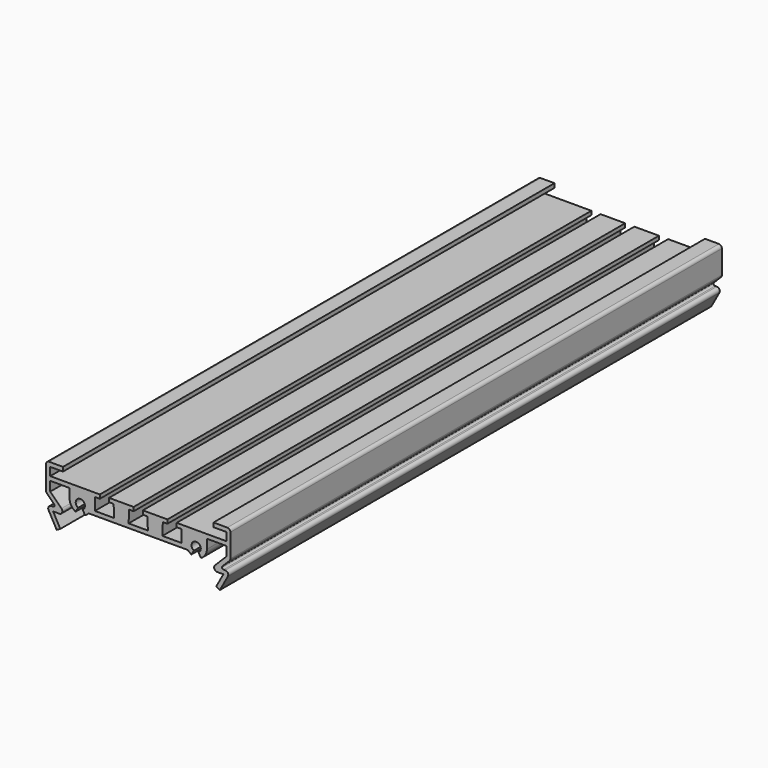
from build123d import *

# Parameters (mm, degrees)
F1_DEPTH = 200


# Not quite as in the source:
# - ends of sketch curves that miss each other by under 0.0002 mm in the source are joined


with BuildPart() as f1:
    # F0 (on Front) → F1 (new body)
    with BuildSketch(Plane.XZ):
        with BuildLine():
            Line((-18.103784, -0.791851), (-17.32476, -2.14116))
            ThreePointArc((-17.32476, -2.14116), (-16.7014064944, -1.7527534112), (-16.1728328101, -1.2428131594))
            Line((-16.1728328101, -1.2428131594), (16.172833, -1.242813))
            ThreePointArc((16.172833, -1.242813), (16.7014064944, -1.7527534112), (17.3247602013, -2.1411595856))
            Line((17.3247602013, -2.1411595856), (18.103784, -0.791851))
            ThreePointArc((18.103784, -0.791851), (18.853784, 2.007187), (19.6037840458, -0.7918510793))
            Line((19.6037840458, -0.7918510793), (20.382808, -2.14116))
            ThreePointArc((20.382808, -2.14116), (21.820396824, -0.8500174455), (22.353784, 1.007187))
            Line((22.353784, 1.007187), (22.353784, 4.007187))
            Line((22.353784, 4.007187), (28.65, 4.007187))
            Line((28.65, 4.007187), (28.65, 0.916375))
            Line((28.65, 0.916375), (24.995488, -2.738136))
            ThreePointArc((24.995488, -2.738136), (24.7787154675, -3.8279264324), (25.702595, -4.445243))
            Line((25.702595, -4.445243), (27.714112, -4.445243))
            Line((27.714112, -4.445243), (25.365346, -8.705386))
            Line((25.365346, -8.705386), (26.54757, -9.357187))
            Line((26.54757, -9.357187), (29.182471, -4.578059))
            ThreePointArc((29.182471, -4.578059), (29.1678006221, -3.5867237514), (28.30675, -3.095243))
            Line((28.30675, -3.095243), (27.754677, -3.095243))
            ThreePointArc((27.754677, -3.095243), (27.292737369, -2.7865850428), (27.4011231094, -2.2416901094))
            Line((27.4011231094, -2.2416901094), (29.707107, 0.064294))
            ThreePointArc((29.707107, 0.064294), (29.9238795325, 0.3887175676), (30, 0.771401))
            Line((30, 0.771401), (30, 8.357187))
            ThreePointArc((30, 8.357187), (29.7071067812, 9.0642937812), (29, 9.357187))
            Line((29, 9.357187), (24.5, 9.357187))
            Line((24.5, 9.357187), (24.5, 8.007187))
            Line((24.5, 8.007187), (28.65, 8.007187))
            Line((28.65, 8.007187), (28.65, 5.357187))
            Line((28.65, 5.357187), (12.5, 5.357187))
            Line((12.5, 5.357187), (12.5, 4.107187))
            Line((12.5, 4.107187), (14, 4.107187))
            Line((14, 4.107187), (14.125, 0.107187))
            Line((14.125, 0.107187), (7.875, 0.107187))
            Line((7.875, 0.107187), (8, 4.107187))
            Line((8, 4.107187), (9.5, 4.107187))
            Line((9.5, 4.107187), (9.5, 5.357187))
            Line((9.5, 5.357187), (1.5, 5.357187))
            Line((1.5, 5.357187), (1.5, 4.107187))
            Line((1.5, 4.107187), (3, 4.107187))
            Line((3, 4.107187), (3.125, 0.107187))
            Line((3.125, 0.107187), (-3.125, 0.107187))
            Line((-3.125, 0.107187), (-3, 4.107187))
            Line((-3, 4.107187), (-1.5, 4.107187))
            Line((-1.5, 4.107187), (-1.5, 5.357187))
            Line((-1.5, 5.357187), (-9.5, 5.357187))
            Line((-9.5, 5.357187), (-9.5, 4.107187))
            Line((-9.5, 4.107187), (-8, 4.107187))
            Line((-8, 4.107187), (-7.875, 0.107187))
            Line((-7.875, 0.107187), (-14.125, 0.107187))
            Line((-14.125, 0.107187), (-14, 4.107187))
            Line((-14, 4.107187), (-12.5, 4.107187))
            Line((-12.5, 4.107187), (-12.5, 5.357187))
            Line((-12.5, 5.357187), (-28.65, 5.357187))
            Line((-28.65, 5.357187), (-28.65, 8.007187))
            Line((-28.65, 8.007187), (-24.5, 8.007187))
            Line((-24.5, 8.007187), (-24.5, 9.357187))
            Line((-24.5, 9.357187), (-29, 9.357187))
            ThreePointArc((-29, 9.357187), (-29.7071067812, 9.0642937812), (-30, 8.357187))
            Line((-30, 8.357187), (-30, 0.771401))
            ThreePointArc((-30, 0.771401), (-29.9238795325, 0.3887175676), (-29.7071067812, 0.0642942188))
            Line((-29.7071067812, 0.0642942188), (-27.401123, -2.24169))
            ThreePointArc((-27.401123, -2.24169), (-27.2927362337, -2.7865847162), (-27.754676, -3.095243))
            Line((-27.754676, -3.095243), (-28.306749, -3.095243))
            ThreePointArc((-28.306749, -3.095243), (-29.1677994994, -3.5867235436), (-29.1824708638, -4.5780589249))
            Line((-29.1824708638, -4.5780589249), (-26.54757, -9.357187))
            Line((-26.54757, -9.357187), (-25.365345, -8.705386))
            Line((-25.365345, -8.705386), (-27.714112, -4.445243))
            Line((-27.714112, -4.445243), (-25.702595, -4.445243))
            ThreePointArc((-25.702595, -4.445243), (-24.7787154675, -3.8279264324), (-24.9954882188, -2.7381362188))
            Line((-24.9954882188, -2.7381362188), (-28.65, 0.916375))
            Line((-28.65, 0.916375), (-28.65, 4.007187))
            Line((-28.65, 4.007187), (-22.353784, 4.007187))
            Line((-22.353784, 4.007187), (-22.353784, 1.007187))
            ThreePointArc((-22.353784, 1.007187), (-21.820396824, -0.8500174455), (-20.3828077987, -2.1411595856))
            Line((-20.3828077987, -2.1411595856), (-19.603784, -0.791851))
            ThreePointArc((-19.603784, -0.791851), (-18.853784, 2.007187), (-18.103784, -0.791851))
        make_face()
    extrude(amount=F1_DEPTH)


solid = f1.part
